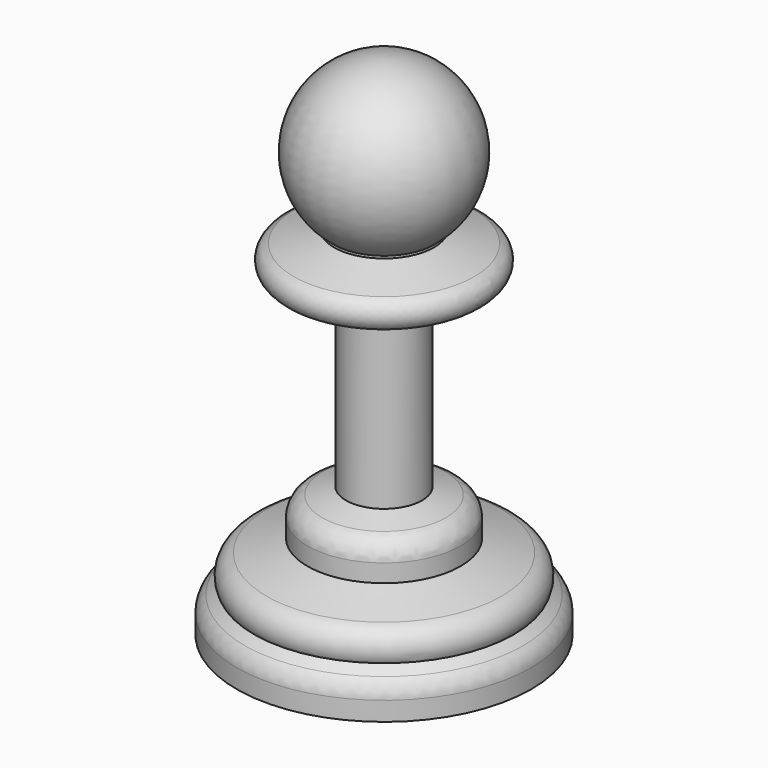
from build123d import *

# Parameters (mm, degrees)
F2_R = 3.6259131904
F4_R = 5.08
F5_R = 5.08


# Not quite as in the source:
# - a fillet or chamfer that OpenCascade refuses, or shapes differently, is made with other operations: its cross-section is extruded or revolved along the edge and cut away or added


with BuildPart() as f1:
    # F0 (on Front) → F1 (revolve)
    with BuildSketch(Plane.XZ):
        with BuildLine():
            Line((0, -74.6885836124), (35.6496162713, -74.6885836124))
            Line((35.6496162713, -74.6885836124), (35.6496162713, -67.5909221172))
            Line((35.6496162713, -67.5909221172), (31.4555428922, -64.3647164106))
            Line((31.4555428922, -64.3647164106), (35.3054043443, -59.3598894102))
            Line((35.3054043443, -59.3598894102), (18.550703302, -54.0408417583))
            Line((18.550703302, -54.0408417583), (18.550703302, -45.9753163159))
            Line((18.550703302, -45.9753163159), (9.1946963221, -43.0717244744))
            Line((9.1946963221, -43.0717244744), (9.1946963221, 0))
            Line((9.1946963221, 0), (37.2865381299, 3.8790097637))
            Line((37.2865381299, 3.8790097637), (12.0982844383, 11.773836799))
            Line((12.0982844383, 11.773836799), (12.0982844383, 12.354565))
            ThreePointArc((12.0982844383, 12.354565), (18.8461202348, 34.6279388467), (0, 48.2829826967))
            Line((0, 48.2829826967), (0, -74.6885836124))
        make_face()
    revolve(axis=Axis((0, 0, -13.2028004579), (0, 0, 1)))

    # F2
    f2_edges = [f1.edges().sort_by_distance(p)[0] for p in [
        (-37.286538, 0, 3.87901),
    ]]
    fillet(f2_edges, radius=F2_R)

    # F3: fillet of radius 5.08 on 1 edges, made by hand

    # F3_s1 → F3_t2 (revolve, cut)
    with BuildSketch(Plane.XZ):
        with BuildLine():
            ThreePointArc((28.4786431175, -57.1926249402), (31.6334069722, -60.0870384375), (31.4555428922, -64.3647164106))
            Line((31.4555428922, -64.3647164106), (35.3054043443, -59.3598894102))
            Line((35.3054043443, -59.3598894102), (28.4786431175, -57.1926249402))
        make_face()
    revolve(axis=Axis((0, 0, -59.3598894102), (0, 0, 1)), mode=Mode.SUBTRACT)

    # F4
    f4_edges = [f1.edges().sort_by_distance(p)[0] for p in [
        (-35.649616, 0, -67.590922),
    ]]
    fillet(f4_edges, radius=F4_R)

    # F5
    f5_edges = [f1.edges().sort_by_distance(p)[0] for p in [
        (-18.550703, 0, -45.975316),
    ]]
    fillet(f5_edges, radius=F5_R)


solid = f1.part
